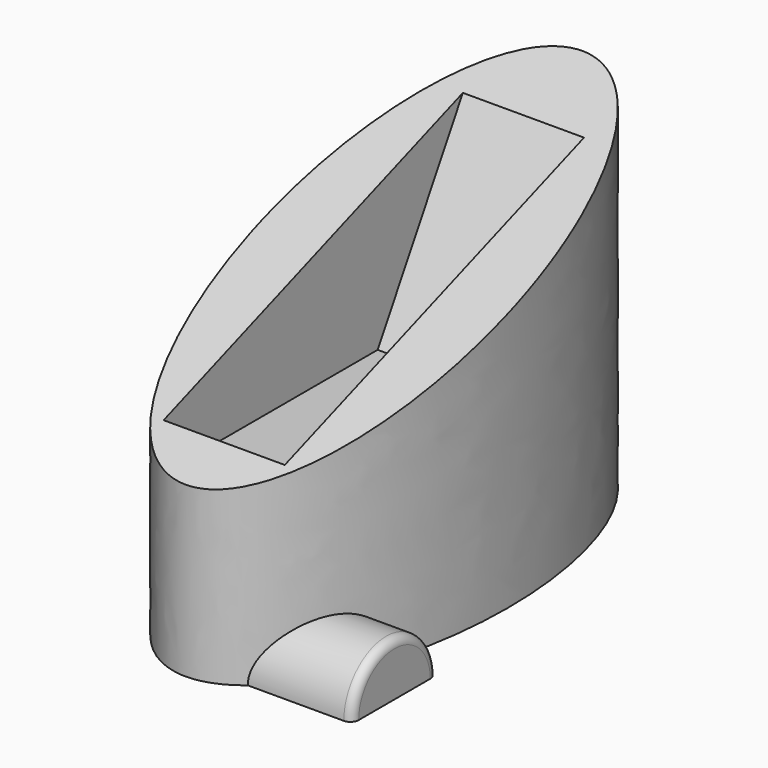
from build123d import *

# Parameters (mm, degrees)
F1_DEPTH = 700
F3_DEPTH = 225
F7_R     = 15
F9_DEPTH = 110


with BuildPart() as f1:
    # F0 (on Top) → F1 (new body)
    with BuildSketch(Plane.XY):
        with BuildLine():
            add(Edge.make_bspline(
                [(0, -450), (389.711431703, -450), (194.8557158515, 225), (0, 900), (-194.8557158515, 225), (-389.711431703, -450), (0, -450)],
                knots=[0, 0, 0, 2.0943951024, 2.0943951024, 4.1887902048, 4.1887902048, 6.2831853072, 6.2831853072, 6.2831853072], degree=2, weights=[1, 0.5, 1, 0.5, 1, 0.5, 1]))
        make_face()
    extrude(amount=F1_DEPTH)

    # F2 (on Right) → F3 (cut, symmetric)
    with BuildSketch(Plane.YZ):
        Polygon((-527.0678045979, 278.585131589), (484.6267700195, 646.8118429184), (306.4921150317, 1136.2327851199), (-705.2024595858, 768.0060737906), align=None)
    extrude(amount=F3_DEPTH, both=True, mode=Mode.SUBTRACT)


with BuildPart() as f6:
    # F5 (on offset) → F6 (new body, up to the next surface of F1)
    with BuildSketch(Plane.YZ.offset(275)):
        with BuildLine():
            Line((-416.1953643573, 0), (-223.8046356427, 0))
            ThreePointArc((-223.8046356427, 0), (-320, 96.1953643573), (-416.1953643573, 0))
        make_face()
    extrude(until=Until.NEXT, target=f1.part, dir=(-1, 0, 0))

    # F7
    f7_edges = [f6.edges().sort_by_distance(p)[0] for p in [
        (275, -320, 96.195364),
    ]]
    fillet(f7_edges, radius=F7_R)


with BuildPart() as f1_1:
    add(f1.part)

    # F8 (on Right) → F9 (cut, symmetric)
    with BuildSketch(Plane.YZ):
        Polygon((123.1035143137, 253.4484267235), (348.1434285641, 640.0269269943), (-362.6262247562, 437.2681677341), (-362.6262247562, 133.130043745), (-302.4670481682, 133.130043745), (-254.562497139, 253.4484267235), align=None)
    extrude(amount=F9_DEPTH, both=True, mode=Mode.SUBTRACT)


solid = Compound([f6.part, f1_1.part])
